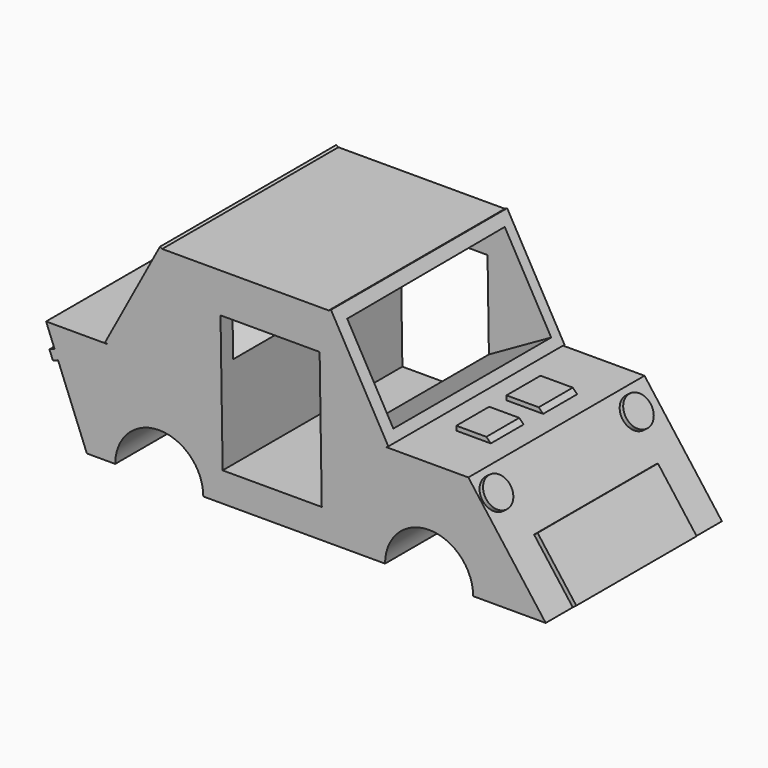
from build123d import *

# Parameters (mm, degrees)
F1_DEPTH    = 30
F2_R        = 4.1236155066
F2_R_2      = 4.1614339228
F2_W        = 4.1973330081
F2_H        = 17.5460492396
F2_W_2      = 4.7969557345
F2_W_3      = 3.5977144726
F2_W_4      = 3.997462336
F2_W_5      = 4.197335802
F2_W_6      = 4.3972060084
F2_W_7      = 3.7975925952
F2_W_8      = 3.3978400752
F2_W_9      = 4.3972097337
F3_DEPTH    = 1.2
F4_W        = 13.7912426144
F4_H        = 11.592639843
F4_W_2      = 13.1916254759
F4_H_2      = 11.1928936094
F5_DEPTH    = 1.2
F6_T4_DEPTH = 37.3094697227
F6_T9_DEPTH = 30.447248054
F8_W        = 60
F8_H        = 31.7812036291
F9_DEPTH    = 0.7
F10_W       = 27.5824870914
F10_H       = 11.8547574278
F10_W_2     = 27.2017772961
F10_H_2     = 2.5796666741
F10_H_3     = 3.0096117407
F11_DEPTH   = 1.5
F12_W       = 60
F12_H       = 31.41779696
F12_W_2     = 52.4410121143
F12_H_2     = 24.1521373391
F13_DEPTH   = 0.7
F15_DEPTH   = 1.2
F16_DEPTH   = 66.4
F17_DEPTH   = 21.8
F18_DEPTH   = 25
F7_W        = 5.1966989413
F7_H        = 17.5460492396
F19_DEPTH   = 2.4
F20_R       = 0.5
F21_DEPTH   = 45.5


# Not quite as in the source:
# - a fillet or chamfer that OpenCascade refuses, or shapes differently, is made with other operations: its cross-section is extruded or revolved along the edge and cut away or added


with BuildPart() as f1:
    # F0 (on Front) → F1 (new body, symmetric)
    with BuildSketch(Plane.XZ):
        Polygon((-39.1735828142, 34.7098528911), (-54.046296189, 7.0353093052), (21.8233727945, 7.0353093052), (6.1976074877, 34.7098528911), align=None)
        with BuildLine():
            Line((-70.8016341305, 7.0353093052), (-59.6941663803, -21.0157584923))
            Line((-59.6941663803, -21.0157584923), (-51.9710250272, -21.0157584923))
            ThreePointArc((-51.9710250272, -21.0157584923), (-39.9710250272, -9.0157584923), (-27.9710250272, -21.0157584923))
            Line((-27.9710250272, -21.0157584923), (21.5446633399, -21.0157584923))
            ThreePointArc((21.5446633399, -21.0157584923), (33.5446633399, -9.0157584923), (45.5446633399, -21.0157584923))
            Line((45.5446633399, -21.0157584923), (65.3119420385, -21.0157584923))
            Line((65.3119420385, -21.0157584923), (44.2265686462, 7.0353093052))
            Line((44.2265686462, 7.0353093052), (21.8233727945, 7.0353093052))
            Line((21.8233727945, 7.0353093052), (-54.046296189, 7.0353093052))
            Line((-54.046296189, 7.0353093052), (-70.8016341305, 7.0353093052))
        make_face()
    extrude(amount=F1_DEPTH, both=True)

    # F2 (on face) → F3 (join)
    with BuildSketch(Plane(origin=(31.6384823097, 0, 23.7819543228), x_dir=(0, 1, 0), z_dir=(0.7993556673, 0, 0.6008581506))):
        with Locations((-25.3838840872, -26.7508905381)):
            Circle(F2_R)
        with Locations((22.3857890815, -26.7508905381)):
            Circle(F2_R_2)
        with Locations((-18.6881348491, -47.2692537384)):
            Rectangle(F2_W, F2_H)
        with Locations((-14.1909904778, -47.2692537384)):
            Rectangle(F2_W_2, F2_H)
        with Locations((-5.9961930383, -47.2692537384)):
            Rectangle(F2_W_3, F2_H)
        with Locations((-9.7937814426, -47.2692537384)):
            Rectangle(F2_W_4, F2_H)
        with Locations((-2.098667901, -47.2692537384)):
            Rectangle(F2_W_5, F2_H)
        with Locations((2.098667901, -47.2692537384)):
            Rectangle(F2_W_5, F2_H)
        with Locations((6.3959388062, -47.2692537384)):
            Rectangle(F2_W_6, F2_H)
        with Locations((10.4933381081, -47.2692537384)):
            Rectangle(F2_W_7, F2_H)
        with Locations((14.0910544433, -47.2692537384)):
            Rectangle(F2_W_8, F2_H)
        with Locations((17.9885793477, -47.2692537384)):
            Rectangle(F2_W_9, F2_H)
    extrude(amount=F3_DEPTH)

    # F4 (on face) → F5 (join)
    with BuildSketch(Plane.XY.offset(7.0353093052)):
        with Locations((35.2776041254, 8.5945435567)):
            Rectangle(F4_W, F4_H)
        with Locations((35.3775396943, -9.1941626742)):
            Rectangle(F4_W_2, F4_H_2)
    extrude(amount=F5_DEPTH)

    # F6: chamfer of 5 on 2 edges, made by hand


with BuildPart() as f6_tool2:
    # F6_s3 → F6_t4 (new body)
    with BuildSketch(Plane.XZ.offset(10.0601913046)):
        Polygon((42.1732254326, 3.2353093052), (37.1732254326, 8.2353093052), (42.1732254326, 8.2353093052), align=None)
    extrude(amount=-F6_T4_DEPTH)

    split(bisect_by=Plane.XY.offset(7.0353093052), keep=Keep.TOP)


with BuildPart() as f1_1:
    add(f1.part)

    # F6_t1: cut F6_tool2
    add(f6_tool2.part, mode=Mode.SUBTRACT)


with BuildPart() as f6_tool7:
    # F6_s8 → F6_t9 (new body)
    with BuildSketch(Plane.XZ.offset(27.6490244188)):
        Polygon((41.9733524323, 3.2353093052), (36.9733524323, 8.2353093052), (41.9733524323, 8.2353093052), align=None)
    extrude(amount=-F6_T9_DEPTH)

    split(bisect_by=Plane.XY.offset(7.0353093052), keep=Keep.TOP)


with BuildPart() as f1_2:
    add(f1_1.part)

    # F6_t6: cut F6_tool7
    add(f6_tool7.part, mode=Mode.SUBTRACT)

    # F8 (on face) → F9 (join)
    with BuildSketch(Plane(origin=(19.559935468, 0, 11.0440470352), x_dir=(0, 1, 0), z_dir=(0.8707833696, 0, 0.4916668824))):
        with Locations((0, 11.2870024924)):
            Rectangle(F8_W, F8_H)
        Polygon((-26.5700668097, -1.8081179587), (-26.5700668097, 23.759579286), (27.1778218448, 23.92606996), (27.1778218448, -1.8081179587), align=None, mode=Mode.SUBTRACT)
    extrude(amount=F9_DEPTH)

    # F10 (on face) → F11 (join)
    with BuildSketch(Plane(origin=(-58.7968134157, 0, -23.2819553802), x_dir=(0, -1, 0), z_dir=(-0.9297621416, 0, -0.3681607801))):
        with Locations((1.9987309352, 8.3647729533)):
            Rectangle(F10_W, F10_H)
        with BuildLine():
            add(Edge.make_bspline(
                [(-4.5523744552, 7.2274826819), (-4.5523744552, 6.5219821956), (-5.2035521005, 6.5219821956)],
                knots=[0, 0, 0, 1, 1, 1], degree=2))
            add(Edge.make_bspline(
                [(-5.2035521005, 6.5219821956), (-5.4103967643, 6.5219821956), (-5.5385429533, 6.5770014833)],
                knots=[0, 0, 0, 1, 1, 1], degree=2))
            Line((-5.5385429533, 6.5770014833), (-5.5385429533, 6.8702055354))
            add(Edge.make_bspline(
                [(-5.5385429533, 6.8702055354), (-5.3881104705, 6.8270258412), (-5.2425531145, 6.8270258412)],
                knots=[0, 0, 0, 1, 1, 1], degree=2))
            add(Edge.make_bspline(
                [(-5.2425531145, 6.8270258412), (-5.0726201247, 6.8270258412), (-4.9932252033, 6.9196532496)],
                knots=[0, 0, 0, 1, 1, 1], degree=2))
            add(Edge.make_bspline(
                [(-4.9932252033, 6.9196532496), (-4.9138302818, 7.012280658), (-4.9138302818, 7.2010177081)],
                knots=[0, 0, 0, 1, 1, 1], degree=2))
            Line((-4.9138302818, 7.2010177081), (-4.9138302818, 9.9784470659))
            Line((-4.9138302818, 9.9784470659), (-4.5523744552, 9.9784470659))
            Line((-4.5523744552, 9.9784470659), (-4.5523744552, 7.2274826819))
        make_face(mode=Mode.SUBTRACT)
        with BuildLine():
            Line((-2.0514344291, 7.5931171887), (-2.3195664007, 7.5931171887))
            Line((-2.3195664007, 7.5931171887), (-2.3913004087, 7.9329831683))
            Line((-2.3913004087, 7.9329831683), (-2.4087115757, 7.9329831683))
            add(Edge.make_bspline(
                [(-2.4087115757, 7.9329831683), (-2.5870019257, 7.7087273375), (-2.7642476056, 7.6289841927)],
                knots=[0, 0, 0, 1, 1, 1], degree=2))
            add(Edge.make_bspline(
                [(-2.7642476056, 7.6289841927), (-2.9414932855, 7.5492410479), (-3.2075359171, 7.5492410479)],
                knots=[0, 0, 0, 1, 1, 1], degree=2))
            add(Edge.make_bspline(
                [(-3.2075359171, 7.5492410479), (-3.5620272769, 7.5492410479), (-3.7633003673, 7.7324065246)],
                knots=[0, 0, 0, 1, 1, 1], degree=2))
            add(Edge.make_bspline(
                [(-3.7633003673, 7.7324065246), (-3.9645734577, 7.9155720013), (-3.9645734577, 8.2526521941)],
                knots=[0, 0, 0, 1, 1, 1], degree=2))
            add(Edge.make_bspline(
                [(-3.9645734577, 8.2526521941), (-3.9645734577, 8.9748674008), (-2.8091684164, 9.0096897347)],
                knots=[0, 0, 0, 1, 1, 1], degree=2))
            Line((-2.8091684164, 9.0096897347), (-2.4045328956, 9.0229222216))
            Line((-2.4045328956, 9.0229222216), (-2.4045328956, 9.1712653644))
            add(Edge.make_bspline(
                [(-2.4045328956, 9.1712653644), (-2.4045328956, 9.4519333762), (-2.5250181712, 9.5856511387)],
                knots=[0, 0, 0, 1, 1, 1], degree=2))
            add(Edge.make_bspline(
                [(-2.5250181712, 9.5856511387), (-2.6455034467, 9.7193689011), (-2.9115460783, 9.7193689011)],
                knots=[0, 0, 0, 1, 1, 1], degree=2))
            add(Edge.make_bspline(
                [(-2.9115460783, 9.7193689011), (-3.2096252571, 9.7193689011), (-3.585706464, 9.5368998711)],
                knots=[0, 0, 0, 1, 1, 1], degree=2))
            Line((-3.585706464, 9.5368998711), (-3.6971379328, 9.8133892029))
            add(Edge.make_bspline(
                [(-3.6971379328, 9.8133892029), (-3.5209369228, 9.908802398), (-3.310958249, 9.963125239)],
                knots=[0, 0, 0, 1, 1, 1], degree=2))
            add(Edge.make_bspline(
                [(-3.310958249, 9.963125239), (-3.1009795751, 10.01744808), (-2.8892597845, 10.01744808)],
                knots=[0, 0, 0, 1, 1, 1], degree=2))
            add(Edge.make_bspline(
                [(-2.8892597845, 10.01744808), (-2.4630344167, 10.01744808), (-2.2572344229, 9.8283628065)],
                knots=[0, 0, 0, 1, 1, 1], degree=2))
            add(Edge.make_bspline(
                [(-2.2572344229, 9.8283628065), (-2.0514344291, 9.639277533), (-2.0514344291, 9.2214095253)],
                knots=[0, 0, 0, 1, 1, 1], degree=2))
            Line((-2.0514344291, 9.2214095253), (-2.0514344291, 7.5931171887))
        make_face(mode=Mode.SUBTRACT)
        with BuildLine():
            Line((2.0938162072, 7.5931171887), (1.7330568272, 7.5931171887))
            Line((1.7330568272, 7.5931171887), (1.7330568272, 9.1448003906))
            add(Edge.make_bspline(
                [(1.7330568272, 9.1448003906), (1.7330568272, 9.4303435291), (1.6111786583, 9.5727668751)],
                knots=[0, 0, 0, 1, 1, 1], degree=2))
            add(Edge.make_bspline(
                [(1.6111786583, 9.5727668751), (1.4893004894, 9.7151902211), (1.2323116647, 9.7151902211)],
                knots=[0, 0, 0, 1, 1, 1], degree=2))
            add(Edge.make_bspline(
                [(1.2323116647, 9.7151902211), (0.8952314718, 9.7151902211), (0.7340040655, 9.5215780442)],
                knots=[0, 0, 0, 1, 1, 1], degree=2))
            add(Edge.make_bspline(
                [(0.7340040655, 9.5215780442), (0.5727766592, 9.3279658673), (0.5727766592, 8.9254196865)],
                knots=[0, 0, 0, 1, 1, 1], degree=2))
            Line((0.5727766592, 8.9254196865), (0.5727766592, 7.5931171887))
            Line((0.5727766592, 7.5931171887), (0.2113208325, 7.5931171887))
            Line((0.2113208325, 7.5931171887), (0.2113208325, 9.1448003906))
            add(Edge.make_bspline(
                [(0.2113208325, 9.1448003906), (0.2113208325, 9.4303435291), (0.0894426636, 9.5727668751)],
                knots=[0, 0, 0, 1, 1, 1], degree=2))
            add(Edge.make_bspline(
                [(0.0894426636, 9.5727668751), (-0.0324355053, 9.7151902211), (-0.2915136701, 9.7151902211)],
                knots=[0, 0, 0, 1, 1, 1], degree=2))
            add(Edge.make_bspline(
                [(-0.2915136701, 9.7151902211), (-0.630683203, 9.7151902211), (-0.7884283759, 9.5118277906)],
                knots=[0, 0, 0, 1, 1, 1], degree=2))
            add(Edge.make_bspline(
                [(-0.7884283759, 9.5118277906), (-0.9461735488, 9.3084653602), (-0.9461735488, 8.8446318717)],
                knots=[0, 0, 0, 1, 1, 1], degree=2))
            Line((-0.9461735488, 8.8446318717), (-0.9461735488, 7.5931171887))
            Line((-0.9461735488, 7.5931171887), (-1.3076293754, 7.5931171887))
            Line((-1.3076293754, 7.5931171887), (-1.3076293754, 9.9784470659))
            Line((-1.3076293754, 9.9784470659), (-1.0137288767, 9.9784470659))
            Line((-1.0137288767, 9.9784470659), (-0.9552273556, 9.6518135732))
            Line((-0.9552273556, 9.6518135732), (-0.9378161886, 9.6518135732))
            add(Edge.make_bspline(
                [(-0.9378161886, 9.6518135732), (-0.8354385267, 9.8259252431), (-0.64913904, 9.9241242249)],
                knots=[0, 0, 0, 1, 1, 1], degree=2))
            add(Edge.make_bspline(
                [(-0.64913904, 9.9241242249), (-0.4628395532, 10.0223232067), (-0.2323157023, 10.0223232067)],
                knots=[0, 0, 0, 1, 1, 1], degree=2))
            add(Edge.make_bspline(
                [(-0.2323157023, 10.0223232067), (0.3269309813, 10.0223232067), (0.4989533112, 9.6169912393)],
                knots=[0, 0, 0, 1, 1, 1], degree=2))
            Line((0.4989533112, 9.6169912393), (0.5163644781, 9.6169912393))
            add(Edge.make_bspline(
                [(0.5163644781, 9.6169912393), (0.6229208201, 9.804335396), (0.8252385805, 9.9133293014)],
                knots=[0, 0, 0, 1, 1, 1], degree=2))
            add(Edge.make_bspline(
                [(0.8252385805, 9.9133293014), (1.0275563409, 10.0223232067), (1.2866345057, 10.0223232067)],
                knots=[0, 0, 0, 1, 1, 1], degree=2))
            add(Edge.make_bspline(
                [(1.2866345057, 10.0223232067), (1.6912700264, 10.0223232067), (1.8925431168, 9.8144338729)],
                knots=[0, 0, 0, 1, 1, 1], degree=2))
            add(Edge.make_bspline(
                [(1.8925431168, 9.8144338729), (2.0938162072, 9.6065445391), (2.0938162072, 9.1489790706)],
                knots=[0, 0, 0, 1, 1, 1], degree=2))
            Line((2.0938162072, 9.1489790706), (2.0938162072, 7.5931171887))
        make_face(mode=Mode.SUBTRACT)
        with BuildLine():
            add(Edge.make_bspline(
                [(-4.8835348513, 10.4429770011), (-4.9444739357, 10.5028714156), (-4.9444739357, 10.6247495845)],
                knots=[0, 0, 0, 1, 1, 1], degree=2))
            add(Edge.make_bspline(
                [(-4.9444739357, 10.6247495845), (-4.9444739357, 10.7487170934), (-4.8835348513, 10.8065221678)],
                knots=[0, 0, 0, 1, 1, 1], degree=2))
            add(Edge.make_bspline(
                [(-4.8835348513, 10.8065221678), (-4.8225957668, 10.8643272422), (-4.7306648051, 10.8643272422)],
                knots=[0, 0, 0, 1, 1, 1], degree=2))
            add(Edge.make_bspline(
                [(-4.7306648051, 10.8643272422), (-4.6436089702, 10.8643272422), (-4.5805805457, 10.8054774978)],
                knots=[0, 0, 0, 1, 1, 1], degree=2))
            add(Edge.make_bspline(
                [(-4.5805805457, 10.8054774978), (-4.5175521212, 10.7466277534), (-4.5175521212, 10.6247495845)],
                knots=[0, 0, 0, 1, 1, 1], degree=2))
            add(Edge.make_bspline(
                [(-4.5175521212, 10.6247495845), (-4.5175521212, 10.5028714156), (-4.5805805457, 10.4429770011)],
                knots=[0, 0, 0, 1, 1, 1], degree=2))
            add(Edge.make_bspline(
                [(-4.5805805457, 10.4429770011), (-4.6436089702, 10.3830825867), (-4.7306648051, 10.3830825867)],
                knots=[0, 0, 0, 1, 1, 1], degree=2))
            add(Edge.make_bspline(
                [(-4.7306648051, 10.3830825867), (-4.8225957668, 10.3830825867), (-4.8835348513, 10.4429770011)],
                knots=[0, 0, 0, 1, 1, 1], degree=2))
        make_face(mode=Mode.SUBTRACT)
        with BuildLine():
            add(Edge.make_bspline(
                [(4.258372487, 7.5854562752), (4.0877430506, 7.5492410479), (3.8460760528, 7.5492410479)],
                knots=[0, 0, 0, 1, 1, 1], degree=2))
            add(Edge.make_bspline(
                [(3.8460760528, 7.5492410479), (3.317473023, 7.5492410479), (3.0113847074, 7.8716958605)],
                knots=[0, 0, 0, 1, 1, 1], degree=2))
            add(Edge.make_bspline(
                [(3.0113847074, 7.8716958605), (2.7052963918, 8.1941506731), (2.7052963918, 8.7659333969)],
                knots=[0, 0, 0, 1, 1, 1], degree=2))
            add(Edge.make_bspline(
                [(2.7052963918, 8.7659333969), (2.7052963918, 9.3432876942), (2.989446637, 9.6828054505)],
                knots=[0, 0, 0, 1, 1, 1], degree=2))
            add(Edge.make_bspline(
                [(2.989446637, 9.6828054505), (3.2735968822, 10.0223232067), (3.7527521977, 10.0223232067)],
                knots=[0, 0, 0, 1, 1, 1], degree=2))
            add(Edge.make_bspline(
                [(3.7527521977, 10.0223232067), (4.2005674126, 10.0223232067), (4.4617349174, 9.727378038)],
                knots=[0, 0, 0, 1, 1, 1], degree=2))
            add(Edge.make_bspline(
                [(4.4617349174, 9.727378038), (4.7229024222, 9.4324328692), (4.7229024222, 8.9490988736)],
                knots=[0, 0, 0, 1, 1, 1], degree=2))
            Line((4.7229024222, 8.9490988736), (4.7229024222, 8.7206643628))
            Line((4.7229024222, 8.7206643628), (3.0799847053, 8.7206643628))
            add(Edge.make_bspline(
                [(3.0799847053, 8.7206643628), (3.0911278522, 8.300707015), (3.2924009426, 8.0830674277)],
                knots=[0, 0, 0, 1, 1, 1], degree=2))
            add(Edge.make_bspline(
                [(3.2924009426, 8.0830674277), (3.493674033, 7.8654278403), (3.8593085397, 7.8654278403)],
                knots=[0, 0, 0, 1, 1, 1], degree=2))
            add(Edge.make_bspline(
                [(3.8593085397, 7.8654278403), (4.2444435534, 7.8654278403), (4.6205247604, 8.0263070233)],
                knots=[0, 0, 0, 1, 1, 1], degree=2))
            Line((4.6205247604, 8.0263070233), (4.6205247604, 7.7038522107))
            add(Edge.make_bspline(
                [(4.6205247604, 7.7038522107), (4.4290019235, 7.6216715025), (4.258372487, 7.5854562752)],
                knots=[0, 0, 0, 1, 1, 1], degree=2))
        make_face(mode=Mode.SUBTRACT)
        with BuildLine():
            add(Edge.make_bspline(
                [(6.7286688592, 8.6377872079), (6.8777084486, 8.481086705), (6.8777084486, 8.2435983873)],
                knots=[0, 0, 0, 1, 1, 1], degree=2))
            add(Edge.make_bspline(
                [(6.8777084486, 8.2435983873), (6.8777084486, 7.9106968745), (6.6297734307, 7.7299689612)],
                knots=[0, 0, 0, 1, 1, 1], degree=2))
            add(Edge.make_bspline(
                [(6.6297734307, 7.7299689612), (6.3818384128, 7.5492410479), (5.9333267512, 7.5492410479)],
                knots=[0, 0, 0, 1, 1, 1], degree=2))
            add(Edge.make_bspline(
                [(5.9333267512, 7.5492410479), (5.4590465625, 7.5492410479), (5.1937003776, 7.6996735306)],
                knots=[0, 0, 0, 1, 1, 1], degree=2))
            Line((5.1937003776, 7.6996735306), (5.1937003776, 8.0346643835))
            add(Edge.make_bspline(
                [(5.1937003776, 8.0346643835), (5.3657227074, 7.9476085485), (5.5624688944, 7.8978126109)],
                knots=[0, 0, 0, 1, 1, 1], degree=2))
            add(Edge.make_bspline(
                [(5.5624688944, 7.8978126109), (5.7592150813, 7.8480166734), (5.942380558, 7.8480166734)],
                knots=[0, 0, 0, 1, 1, 1], degree=2))
            add(Edge.make_bspline(
                [(5.942380558, 7.8480166734), (6.2251379099, 7.8480166734), (6.3773115094, 7.9382065183)],
                knots=[0, 0, 0, 1, 1, 1], degree=2))
            add(Edge.make_bspline(
                [(6.3773115094, 7.9382065183), (6.5294851088, 8.0283963633), (6.5294851088, 8.2136511801)],
                knots=[0, 0, 0, 1, 1, 1], degree=2))
            add(Edge.make_bspline(
                [(6.5294851088, 8.2136511801), (6.5294851088, 8.352940516), (6.4089998333, 8.4518359445)],
                knots=[0, 0, 0, 1, 1, 1], degree=2))
            add(Edge.make_bspline(
                [(6.4089998333, 8.4518359445), (6.2885145577, 8.550731373), (5.9375054313, 8.6858420288)],
                knots=[0, 0, 0, 1, 1, 1], degree=2))
            add(Edge.make_bspline(
                [(5.9375054313, 8.6858420288), (5.6046039185, 8.8098095377), (5.4642699126, 8.9024369461)],
                knots=[0, 0, 0, 1, 1, 1], degree=2))
            add(Edge.make_bspline(
                [(5.4642699126, 8.9024369461), (5.3239359066, 8.9950643545), (5.2553359087, 9.11241562)],
                knots=[0, 0, 0, 1, 1, 1], degree=2))
            add(Edge.make_bspline(
                [(5.2553359087, 9.11241562), (5.1867359108, 9.2297668855), (5.1867359108, 9.3927354085)],
                knots=[0, 0, 0, 1, 1, 1], degree=2))
            add(Edge.make_bspline(
                [(5.1867359108, 9.3927354085), (5.1867359108, 9.6845465672), (5.4242242285, 9.8534348869)],
                knots=[0, 0, 0, 1, 1, 1], degree=2))
            add(Edge.make_bspline(
                [(5.4242242285, 9.8534348869), (5.6617125462, 10.0223232067), (6.0747054271, 10.0223232067)],
                knots=[0, 0, 0, 1, 1, 1], degree=2))
            add(Edge.make_bspline(
                [(6.0747054271, 10.0223232067), (6.4598404409, 10.0223232067), (6.8282607343, 9.8656227038)],
                knots=[0, 0, 0, 1, 1, 1], degree=2))
            Line((6.8282607343, 9.8656227038), (6.6994180986, 9.5717222051))
            add(Edge.make_bspline(
                [(6.6994180986, 9.5717222051), (6.3407480587, 9.7193689011), (6.0489369, 9.7193689011)],
                knots=[0, 0, 0, 1, 1, 1], degree=2))
            add(Edge.make_bspline(
                [(6.0489369, 9.7193689011), (5.7919480753, 9.7193689011), (5.6613643229, 9.6389293097)],
                knots=[0, 0, 0, 1, 1, 1], degree=2))
            add(Edge.make_bspline(
                [(5.6613643229, 9.6389293097), (5.5307805705, 9.5584897182), (5.5307805705, 9.4171110422)],
                knots=[0, 0, 0, 1, 1, 1], degree=2))
            add(Edge.make_bspline(
                [(5.5307805705, 9.4171110422), (5.5307805705, 9.3210014005), (5.5798800614, 9.2537942959)],
                knots=[0, 0, 0, 1, 1, 1], degree=2))
            add(Edge.make_bspline(
                [(5.5798800614, 9.2537942959), (5.6289795523, 9.1865871913), (5.7376252343, 9.1256481069)],
                knots=[0, 0, 0, 1, 1, 1], degree=2))
            add(Edge.make_bspline(
                [(5.7376252343, 9.1256481069), (5.8462709163, 9.0647090224), (6.155493242, 8.9490988736)],
                knots=[0, 0, 0, 1, 1, 1], degree=2))
            add(Edge.make_bspline(
                [(6.155493242, 8.9490988736), (6.5796292698, 8.7944877108), (6.7286688592, 8.6377872079)],
                knots=[0, 0, 0, 1, 1, 1], degree=2))
        make_face(mode=Mode.SUBTRACT)
        with Locations((16.3991113519, 25.0407643616)):
            Rectangle(F10_W_2, F10_H_2)
        with Locations((-16.3991113519, 25.2557368949)):
            Rectangle(F10_W_2, F10_H_3)
    extrude(amount=F11_DEPTH)

    # F12 (on face) → F13 (join)
    with BuildSketch(Plane(origin=(-44.8684911382, 0, 24.1129977875), x_dir=(0, -1, 0), z_dir=(-0.880855638, 0, 0.473384986))):
        with Locations((0, -3.6787148195)):
            Rectangle(F12_W, F12_H)
        with Locations((-0.2835597843, -4.0873009712)):
            Rectangle(F12_W_2, F12_H_2, mode=Mode.SUBTRACT)
    extrude(amount=F13_DEPTH)

    # F14 (on face) → F15 (join)
    with BuildSketch(Plane(origin=(0, 30, 0), x_dir=(-1, 0, 0), z_dir=(0, 1, 0))):
        Polygon((26.2039810535, 25.5836990518), (-5.4300072668, 25.5836990518), (-6.0798813504, -15.8031989677), (25.5541069699, -15.8031989677), align=None)
        Polygon((-4.3003342153, -13.0384113724), (-3.7194166203, 23.9570280053), (23.2805833797, 23.9570280053), (22.6996657847, -13.0384113724), align=None, mode=Mode.SUBTRACT)
    extrude(amount=F15_DEPTH)

    # F14 (on face) → F16 (cut)
    with BuildSketch(Plane(origin=(0, 30, 0), x_dir=(-1, 0, 0), z_dir=(0, 1, 0))):
        Polygon((23.2805833797, 23.9570280053), (-3.7194166203, 23.9570280053), (-4.3003342153, -13.0384113724), (22.6996657847, -13.0384113724), align=None)
    extrude(amount=-F16_DEPTH, mode=Mode.SUBTRACT)

    # F8 (on face) → F17 (cut)
    with BuildSketch(Plane(origin=(19.559935468, 0, 11.0440470352), x_dir=(0, 1, 0), z_dir=(0.8707833696, 0, 0.4916668824))):
        Polygon((27.1778218448, 23.92606996), (-26.5700668097, 23.759579286), (-26.5700668097, -1.8081179587), (27.1778218448, -1.8081179587), align=None)
    extrude(amount=-F17_DEPTH, mode=Mode.SUBTRACT)

    # F12 (on face) → F18 (cut)
    with BuildSketch(Plane(origin=(-44.8684911382, 0, 24.1129977875), x_dir=(0, -1, 0), z_dir=(-0.880855638, 0, 0.473384986))):
        with Locations((-0.2835597843, -4.0873009712)):
            Rectangle(F12_W_2, F12_H_2)
    extrude(amount=-F18_DEPTH, mode=Mode.SUBTRACT)

    # F7 (on face) → F19 (join)
    with BuildSketch(Plane(origin=(32.5977091105, 0, 24.5029841035), x_dir=(0, 1, 0), z_dir=(0.7993556673, 0, 0.6008581506))):
        Polygon((-0.2998085693, -38.4962291186), (-6.3959406689, -38.4962291186), (-6.3959406689, -56.0422783582), (0, -56.0422783582), align=None)
        Polygon((11.1928945407, -38.4962291186), (5.5964454077, -38.4962291186), (5.896253977, -56.0422783582), (11.1928945407, -56.0422783582), align=None)
        with Locations((-14.1909900121, -47.2692537384)):
            Rectangle(F7_W, F7_H)
    extrude(amount=-F19_DEPTH)

    # F20 (on face) → F21 (cut)
    with BuildSketch(Plane.XY.offset(25.5836990518)):
        with Locations((3.6855896469, 30.619546771)):
            Circle(F20_R)
    extrude(amount=-F21_DEPTH, mode=Mode.SUBTRACT)


solid = f1_2.part
